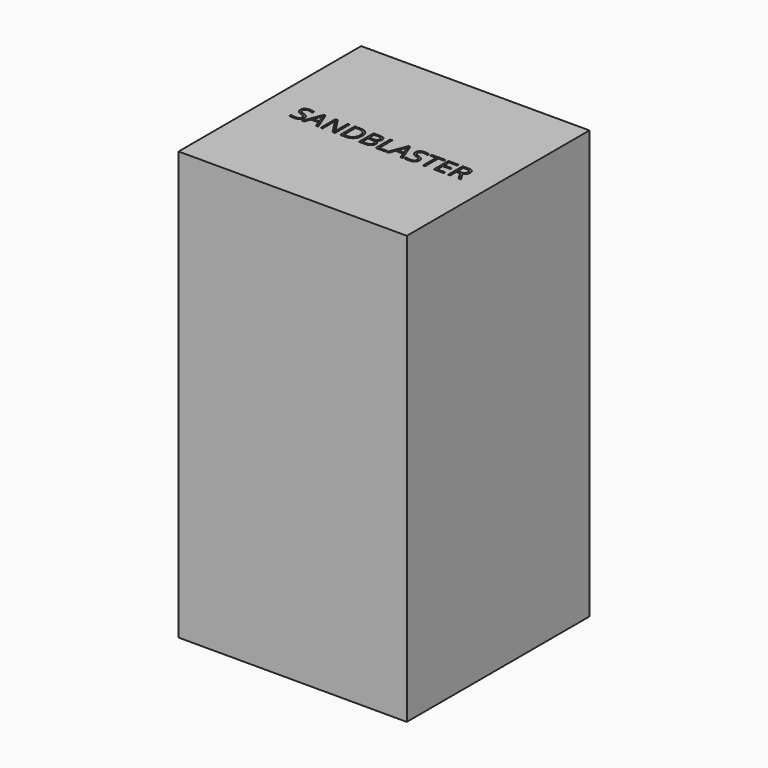
from build123d import *

# Parameters (mm, degrees)
F0_W         = 800
F0_H         = 800
F1_DEPTH     = 1500
F2_TEXT_SIZE = 90.310814607
F3_DEPTH     = 25


# Not quite as in the source:
# - Text() gives the source's letters only with a copy of the font that has no kerning and outlines rounded to 1/6400 em; it was checked with that copy


with BuildPart() as f1:
    # F0 (on Top) → F1 (new body)
    with BuildSketch(Plane.XY):
        Rectangle(F0_W, F0_H)
    extrude(amount=F1_DEPTH)

    # F2 (on face) → F3 (cut)
    with BuildSketch(Plane.XY.offset(1500)):
        with Locations((-300, -46.9229340366)):
            Text('SANDBLASTER', F2_TEXT_SIZE, font='Open Sans', text_align=(TextAlign.LEFT, TextAlign.BOTTOM))
    extrude(amount=-F3_DEPTH, mode=Mode.SUBTRACT)


solid = f1.part
